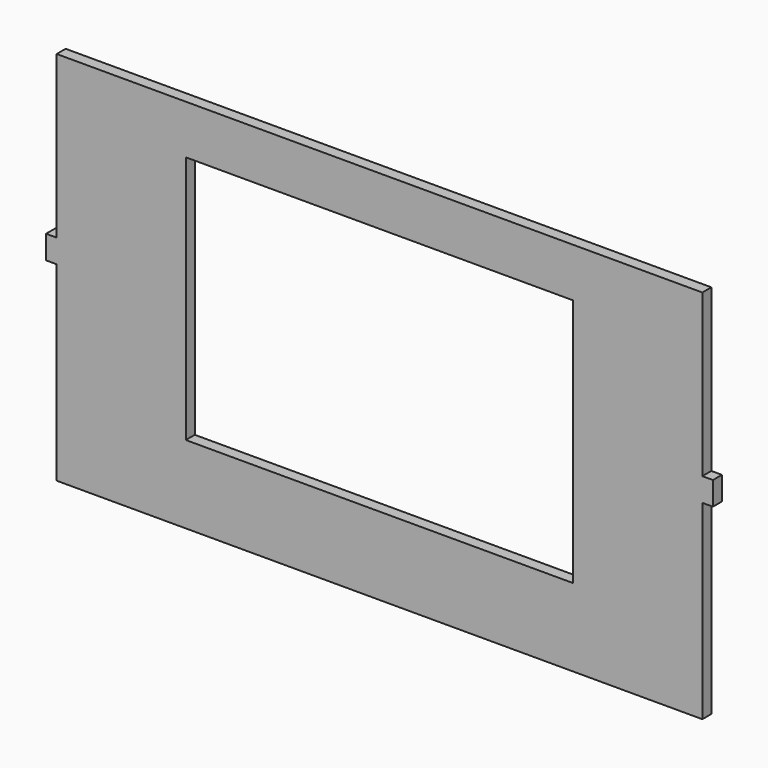
from build123d import *

# Parameters (mm, degrees)
F1_DEPTH = 4.8


# Not quite as in the source:
# - a feature names something its author has since deleted; it is built from what else it names


with BuildPart() as f1:
    # F0 (on Front) → F1 (new body)
    with BuildSketch(Plane.XZ):
        Polygon((-36.6599317901, 103.4564594077), (-174.1599317901, 103.4564594077), (-174.1599317901, 34.6020694077), (-174.1599317901, 29.6020694077), (-174.1599317901, 24.6020694077), (-174.1599317901, -56.5435405923), (-36.6599317901, -56.5435405923), (-36.6599317901, -23.3979305923), (-119.1599317901, -23.3979305923), (-119.1599317901, 82.6020694077), (-36.6599317901, 82.6020694077), align=None)
        Polygon((100.8400682099, 103.4564594077), (-36.6599317901, 103.4564594077), (-36.6599317901, 82.6020694077), (45.8400682099, 82.6020694077), (45.8400682099, -23.3979305923), (-36.6599317901, -23.3979305923), (-36.6599317901, -56.5435405923), (100.8400682099, -56.5435405923), (100.8400682099, 24.6020694077), (100.8400682099, 29.6020694077), (100.8400682099, 34.6020694077), align=None)
        Polygon((105.3400682099, 34.6020694077), (100.8400682099, 34.6020694077), (100.8400682099, 29.6020694077), (101.9359001704, 29.6020694077), (105.3400682099, 29.6020694077), align=None)
        Polygon((101.9359001704, 29.6020694077), (100.8400682099, 29.6020694077), (100.8400682099, 24.6020694077), (101.9359001704, 24.6020694077), (105.3400682099, 24.6020694077), (105.3400682099, 29.6020694077), align=None)
        Polygon((-174.1599317901, 29.6020694077), (-174.1599317901, 34.6020694077), (-178.6599317901, 34.6020694077), (-178.6599317901, 29.6020694077), (-175.2557637506, 29.6020694077), align=None)
        Polygon((-174.1599317901, 24.6020694077), (-174.1599317901, 29.6020694077), (-175.2557637506, 29.6020694077), (-178.6599317901, 29.6020694077), (-178.6599317901, 24.6020694077), (-175.2557637506, 24.6020694077), align=None)
    extrude(amount=F1_DEPTH)


solid = f1.part
